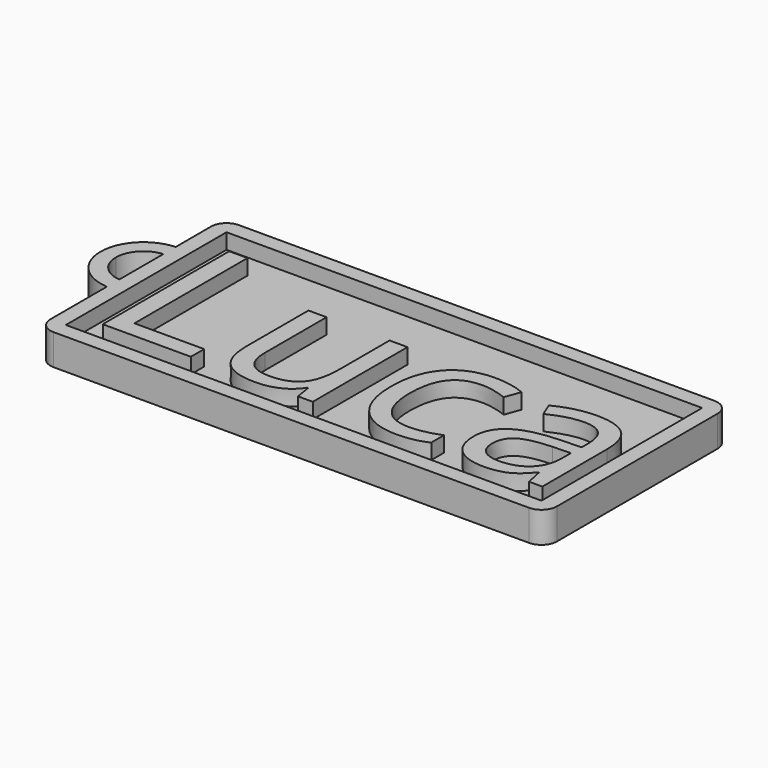
from build123d import *

# Parameters (mm, degrees)
F0_W         = 61.5714335345
F0_H         = 26
F1_DEPTH     = 2
F2_DEPTH     = 4
F3_TEXT_SIZE = 28.6524521647
F4_DEPTH     = 2
F6_DEPTH     = 4


# Not quite as in the source:
# - Text() gives the source's letters only with a copy of the font that has no kerning and outlines rounded to 1/6400 em; it was checked with that copy


with BuildPart() as f1:
    # F0 (on Top) → F1 (new body)
    with BuildSketch(Plane.XY):
        with Locations((0, -1.7142857372)):
            Rectangle(F0_W, F0_H)
    extrude(amount=F1_DEPTH)

    # F0 (on Top) → F2 (join)
    with BuildSketch(Plane.XY):
        with BuildLine():
            ThreePointArc((32.7857167672, 11.2857142628), (32.1999303296, 12.6999278252), (30.7857167672, 13.2857142628))
            Line((30.7857167672, 13.2857142628), (-30.7857167672, 13.2857142628))
            ThreePointArc((-30.7857167672, 13.2857142628), (-32.1999303296, 12.6999278252), (-32.7857167672, 11.2857142628))
            Line((-32.7857167672, 11.2857142628), (-32.7857167672, -14.7142857372))
            ThreePointArc((-32.7857167672, -14.7142857372), (-32.1999303296, -16.1284992995), (-30.7857167672, -16.7142857372))
            Line((-30.7857167672, -16.7142857372), (30.7857167672, -16.7142857372))
            ThreePointArc((30.7857167672, -16.7142857372), (32.1999303296, -16.1284992995), (32.7857167672, -14.7142857372))
            Line((32.7857167672, -14.7142857372), (32.7857167672, 11.2857142628))
        make_face()
        with Locations((0, -1.7142857372)):
            Rectangle(F0_W, F0_H, mode=Mode.SUBTRACT)
    extrude(amount=F2_DEPTH)

    # F3 (on face) → F4 (join)
    with BuildSketch(Plane.XY.offset(2)):
        with Locations((-30.7857167672, -12.2552599924)):
            Text('Luca', F3_TEXT_SIZE, font='Open Sans', text_align=(TextAlign.LEFT, TextAlign.BOTTOM))
    extrude(amount=F4_DEPTH)

    # F5 (on Top) → F6 (join)
    with BuildSketch(Plane.XY):
        with BuildLine():
            ThreePointArc((-32.5034633279, 5.5717462016), (-36.4432828501, 3.9398195222), (-38.0752095295, 0))
            ThreePointArc((-38.0752095295, 0), (-36.4432828501, -3.9398195222), (-32.5034633279, -5.5717462016))
            Line((-32.5034633279, -5.5717462016), (-32.5034633279, -3.5717462016))
            ThreePointArc((-32.5034633279, -3.5717462016), (-35.0290692877, -2.5256059598), (-36.0752095295, 0))
            ThreePointArc((-36.0752095295, 0), (-35.0290692877, 2.5256059598), (-32.5034633279, 3.5717462016))
            Line((-32.5034633279, 3.5717462016), (-32.5034633279, 5.5717462016))
        make_face()
    extrude(amount=F6_DEPTH)


solid = f1.part
